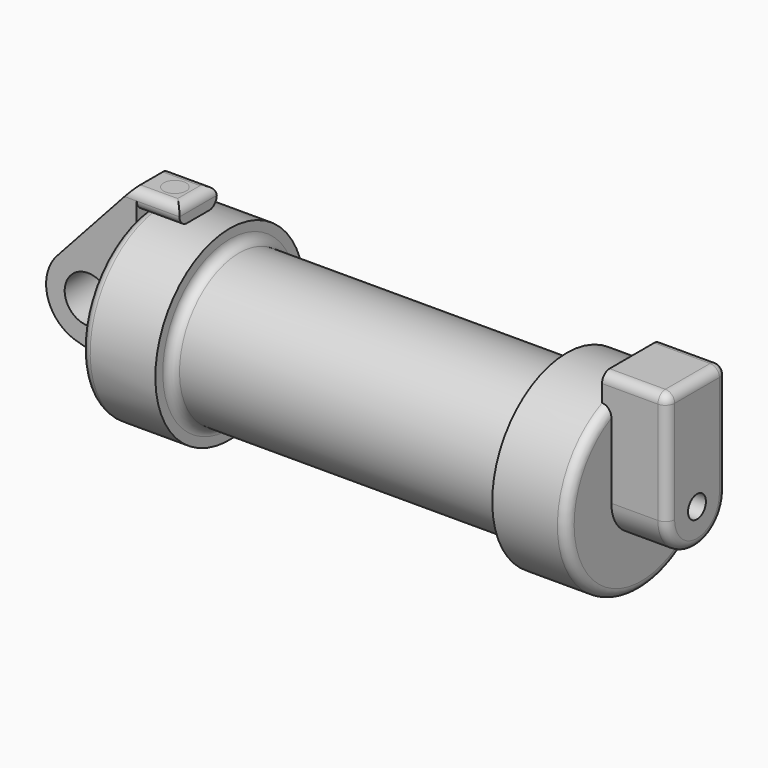
from build123d import *

# Parameters (mm, degrees)
F0_W          = 5.842
F0_H          = 12.7
F0_R          = 3.175
F2_DEPTH      = 3.175
F3_R          = 1.524
F4_DEPTH      = 7.62
F4_DEPTH_BACK = 1.27
F7_R          = 1.524
F8_DEPTH      = 17.78
F9_R          = 1.27
F10_R         = 1.27
F11_T1_DEPTH  = 15.24
F12_R         = 1.26999
F12_2_R       = 1.26999
F13_R         = 1.27


# Not quite as in the source:
# - a fillet or chamfer that OpenCascade refuses, or shapes differently, is made with other operations: its cross-section is extruded or revolved along the edge and cut away or added
# - a fillet or chamfer is up to 0.001 mm smaller than in the source, because OpenCascade refuses the exact size
# - the program builds the solid bodies; features that only make, move or delete a surface that nothing else refers to are left out


with BuildPart() as f1:
    # F0 (on Front) → F1 (revolve)
    with BuildSketch(Plane.XZ):
        Polygon((5.842, 12.7), (5.842, 0), (66.294, 0), (66.294, 12.7), (56.134, 12.7), (56.134, 10.16), (10.16, 10.16), (10.16, 12.7), align=None)
        with Locations((2.921, 6.35)):
            Rectangle(F0_W, F0_H)
    revolve(axis=Axis((33.147, 0, 0), (-1, 0, 0)))

    # F3 (on face) → F4 (join, two sides)
    with BuildSketch(Plane.YZ.offset(66.294)) as f4_sk:
        with BuildLine():
            ThreePointArc((-5.08, 0), (0, -5.08), (5.08, 0))
            ThreePointArc((5.08, 0), (0, 5.08), (-5.08, 0))
        make_face()
        Circle(F3_R, mode=Mode.SUBTRACT)
        with BuildLine():
            ThreePointArc((-5.08, 0), (0, 5.08), (5.08, 0))
            Line((5.08, 0), (5.08, 15.24))
            Line((5.08, 15.24), (-5.08, 15.24))
            Line((-5.08, 15.24), (-5.08, 0))
        make_face()
    extrude(amount=F4_DEPTH)
    extrude(f4_sk.sketch, amount=-F4_DEPTH_BACK)

    # F9
    f9_edges = [f1.edges().sort_by_distance(p)[0] for p in [
        (10.16, 0, -10.16),
    ]]
    fillet(f9_edges, radius=F9_R)

    # F10
    f10_edges = [f1.edges().sort_by_distance(p)[0] for p in [
        (56.134, 0, -10.16),
    ]]
    fillet(f10_edges, radius=F10_R)

    # F11: fillet of radius 1.27 on 1 edges, made by hand

    # F11_s2 → F11_t1 (cut)
    with BuildSketch(Plane.YZ.offset(61.849)):
        with BuildLine():
            ThreePointArc((-5.08, 13.97), (-4.7080256121, 14.8680256121), (-3.81, 15.24))
            Line((-3.81, 15.24), (-5.08, 15.24))
            Line((-5.08, 15.24), (-5.08, 13.97))
        make_face()
    extrude(amount=F11_T1_DEPTH, mode=Mode.SUBTRACT)

    # F12 (radius 1.27 in the source; OpenCascade refuses exactly that, so slightly less here)
    f12_edges = [f1.edges().sort_by_distance(p)[0] for p in [
        (73.914, 0.635, 15.24),
        (69.469, 5.08, 15.24),
        (66.294, 0, -12.7),
    ]]
    fillet(f12_edges, radius=F12_R)

    # F13
    f13_edges = [f1.edges().sort_by_distance(p)[0] for p in [
        (0, 0, -12.7),
    ]]
    fillet(f13_edges, radius=F13_R)


with BuildPart() as f2:
    # F0 (on Front) → F2 (new body, symmetric)
    with BuildSketch(Plane.XZ):
        with BuildLine():
            Line((-0.9398, 0), (0, 0))
            Line((0, 0), (0, 12.7))
            Line((0, 12.7), (5.842, 12.7))
            Line((5.842, 12.7), (5.842, 15.24))
            Line((5.842, 15.24), (-0.508, 15.24))
            Line((-0.508, 15.24), (-10.8806298187, 3.8475430269))
            ThreePointArc((-10.8806298187, 3.8475430269), (-4.5919612295, 5.3297205562), (-0.9398, 0))
        make_face()
        with BuildLine():
            ThreePointArc((-8.1826630726, -5.5069827884), (-3.1957909266, -4.5493385486), (-0.9398, 0))
            ThreePointArc((-0.9398, 0), (-4.5919612295, 5.3297205562), (-10.8806298187, 3.8475430269))
            ThreePointArc((-10.8806298187, 3.8475430269), (-12.1459778134, -1.5837270034), (-8.1826630726, -5.5069827884))
        make_face()
        with Locations((-6.6548, 0)):
            Circle(F0_R, mode=Mode.SUBTRACT)
        with BuildLine():
            Line((5.842, 0), (0, 0))
            Line((0, 0), (-0.9398, 0))
            ThreePointArc((-0.9398, 0), (-3.1957909266, -4.5493385486), (-8.1826630726, -5.5069827884))
            Line((-8.1826630726, -5.5069827884), (5.842, -9.398))
            Line((5.842, -9.398), (5.842, 0))
        make_face()
    extrude(amount=F2_DEPTH, both=True)

    # F12#2 (radius 1.27 in the source; OpenCascade refuses exactly that, so slightly less here)
    f12_2_edges = [f2.edges().sort_by_distance(p)[0] for p in [
        (2.667, -3.175, 15.24),
        (2.921, -3.175, 12.7),
        (2.667, 3.175, 15.24),
        (2.921, 3.175, 12.7),
        (5.842, 0, 15.24),
    ]]
    fillet(f12_2_edges, radius=F12_2_R)


with BuildPart() as f8:
    # F7 (on face) → F8 (new body)
    with BuildSketch(Plane.XY.offset(15.24)):
        with Locations((2.667, 0)):
            Circle(F7_R)
    extrude(amount=-F8_DEPTH)


solid = Compound([f1.part, f2.part, f8.part])
